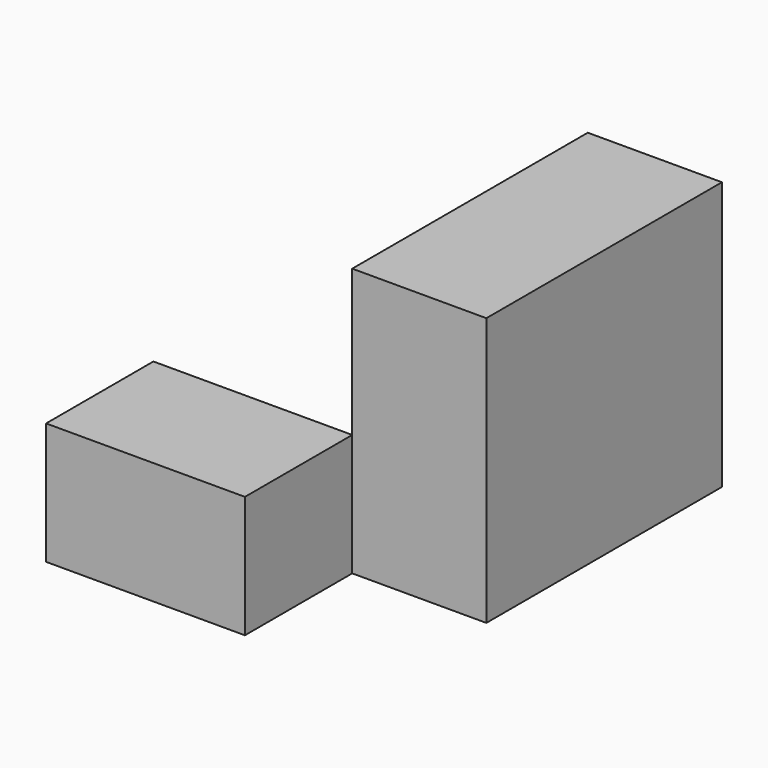
from build123d import *

# Parameters (mm, degrees)
F0_W     = 55.7560741802
F0_H     = 50.8
F1_DEPTH = 25.4
F2_W     = 37.6538187265
F2_H     = 23.0797566473
F3_DEPTH = 25.4


# Not quite as in the source:
# - ends of sketch curves that miss each other by under 0.0002 mm in the source are joined


with BuildPart() as f1:
    # F0 (on Right) → F1 (new body)
    with BuildSketch(Plane.YZ):
        with Locations((27.8780370901, 25.4)):
            Rectangle(F0_W, F0_H)
    extrude(amount=F1_DEPTH)


with BuildPart() as f3:
    # F2 (on face) → F3 (new body)
    with BuildSketch(Plane.XZ):
        with Locations((-18.8269093633, 11.5398783237)):
            Rectangle(F2_W, F2_H)
    extrude(amount=F3_DEPTH)


solid = Compound([f1.part, f3.part])
